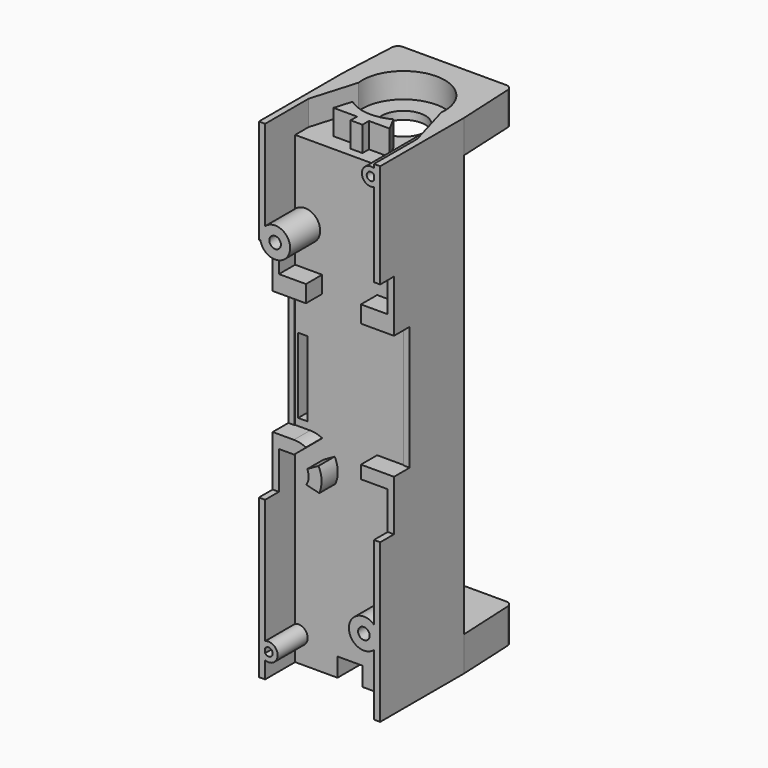
from build123d import *

# Parameters (mm, degrees)
F1_W           = 19.4
F1_H           = 5.4
F1_W_2         = 13
F1_H_2         = 3.4
F1_H_3         = 67.45
F1_R           = 2.4
F1_R_2         = 1.75
F2_DEPTH       = 13.5
F4_START       = -10
F4_DEPTH       = 17
F5_W           = 13
F5_H           = 3.4
F6_DEPTH       = 2.1
F7_DEPTH       = 2.25
F8_R           = 3.5
F9_DEPTH       = 7.5
F10_R          = 2
F11_DEPTH      = 7.5
F12_R          = 3.5
F13_DEPTH      = 4
F12_W          = 17.4
F12_H          = 6
F14_DEPTH      = 80
F15_W          = 3.989465184
F15_H          = 1.1423683461
F16_DEPTH      = 3
F17_W          = 2.7596634789
F17_H          = 19.85
F17_H_2        = 8.35
F17_W_2        = 3.1403365211
F17_H_3        = 8.1
F18_DEPTH      = 20
F19_W          = 1
F19_H          = 2.0696715653
F19_W_2        = 3.1403365211
F20_DEPTH      = 18.4
F21_DEPTH      = 25
F22_DEPTH      = 13.5
F23_W          = 8.7971314788
F23_H          = 3.2557382435
F24_DEPTH      = 80
F25_R          = 1.425
F25_R_2        = 0.65
F25_R_3        = 1.45
F26_DEPTH      = 21
F26_DEPTH_BACK = 6
F27_R          = 1.75
F27_R_2        = 0.925
F27_R_3        = 1.8673061799
F28_DEPTH      = 2.75
F29_W          = 1.5
F29_H          = 12
F30_DEPTH      = 21.001
F31_DEPTH      = 33.725
F32_R          = 6.2849648465
F33_DEPTH      = 2
F35_DEPTH      = 3.2403365211
F36_DEPTH      = 3.2403365211
F38_DEPTH      = 78.251


with BuildPart() as f2:
    # F1 (on Front) → F2 (new body, symmetric)
    with BuildSketch(Plane.XZ):
        with Locations((0, 75.55)):
            Rectangle(F1_W, F1_H)
        with Locations((0, 75.55)):
            Rectangle(F1_W_2, F1_H_2, mode=Mode.SUBTRACT)
        with Locations((0, 39.125)):
            Rectangle(F1_W, F1_H_3)
        with Locations((7.1, 11.6)):
            Circle(F1_R, mode=Mode.SUBTRACT)
        with Locations((-7.1, 62.05)):
            Circle(F1_R, mode=Mode.SUBTRACT)
        with Locations((-7.1, 62.05)):
            Circle(F1_R)
        with Locations((-7.1, 62.05)):
            Circle(F1_R_2, mode=Mode.SUBTRACT)
        with Locations((7.1, 11.6)):
            Circle(F1_R)
        with Locations((7.1, 11.6)):
            Circle(F1_R_2, mode=Mode.SUBTRACT)
        with Locations((0, 2.7)):
            Rectangle(F1_W, F1_H)
        with Locations((0, 2.7)):
            Rectangle(F1_W_2, F1_H_2, mode=Mode.SUBTRACT)
        with Locations((0, 2.7)):
            Rectangle(F1_W_2, F1_H_2)
        with Locations((0, 75.55)):
            Rectangle(F1_W_2, F1_H_2)
    extrude(amount=F2_DEPTH, both=True)

    # F1 (on Front) → F4 (cut)
    with BuildSketch(Plane.XZ.offset(F4_START)):
        with Locations((0, 2.7)):
            Rectangle(F1_W_2, F1_H_2)
        with Locations((0, 75.55)):
            Rectangle(F1_W_2, F1_H_2)
    extrude(amount=-F4_DEPTH, mode=Mode.SUBTRACT)

    # F5 (on face) → F6 (join)
    with BuildSketch(Plane(origin=(0, 13.5, 0), x_dir=(-1, 0, 0), z_dir=(0, 1, 0))):
        with Locations((0, 75.55)):
            Rectangle(F5_W, F5_H)
        with Locations((0, 2.7)):
            Rectangle(F5_W, F5_H)
    extrude(amount=-F6_DEPTH)

    # F5 (on face) → F7 (cut)
    with BuildSketch(Plane(origin=(0, 13.5, 0), x_dir=(-1, 0, 0), z_dir=(0, 1, 0))):
        with Locations((0, 75.55)):
            Rectangle(F5_W, F5_H)
        with Locations((0, 2.7)):
            Rectangle(F5_W, F5_H)
    extrude(amount=-F7_DEPTH, mode=Mode.SUBTRACT)

    # F8 (on face) → F9 (cut, symmetric)
    with BuildSketch(Plane.XY.offset(78.25)):
        with Locations((0, 3.3)):
            Circle(F8_R)
    extrude(amount=F9_DEPTH, both=True, mode=Mode.SUBTRACT)

    # F10 (on face) → F11 (cut, symmetric)
    with BuildSketch(Plane(origin=(0, 0, 0), x_dir=(1, 0, 0), z_dir=(0, 0, -1))):
        with Locations((0, -3.3)):
            Circle(F10_R)
    extrude(amount=F11_DEPTH, both=True, mode=Mode.SUBTRACT)

    # F12 (on face) → F13 (cut)
    with BuildSketch(Plane.XY.offset(78.25)):
        with BuildLine():
            Line((-6.5448551873, 2.4486066849), (-8.7, -4.8))
            Line((-8.7, -4.8), (-4.7295154072, -4.8))
            Line((-4.7295154072, -4.8), (-3.9035302168, -2.0218842383))
            ThreePointArc((-3.9035302168, -2.0218842383), (-5.6822980969, -0.0573037304), (-6.5448551873, 2.4486066849))
        make_face()
        with BuildLine():
            Line((8.7, -4.8), (6.5659687916, 2.6306317698))
            ThreePointArc((6.5659687916, 2.6306317698), (5.4611174799, -0.4062374277), (3.0469932229, -2.5545565417))
            Line((3.0469932229, -2.5545565417), (4.2667957023, -4.8))
            Line((4.2667957023, -4.8), (8.7, -4.8))
        make_face()
        Polygon((-4.7295154072, -4.8), (-8.7, -4.8), (-8.7, -7.5), (8.7, -7.5), (8.7, -4.8), (4.2667957023, -4.8), (0.95, -4.8), (0.95, -6.1), (-0.95, -6.1), (-0.95, -4.8), align=None)
        with BuildLine():
            ThreePointArc((6.6, 3.3), (-0.4265886565, 9.8861993682), (-6.5448551873, 2.4486066849))
            ThreePointArc((-6.5448551873, 2.4486066849), (-5.6822980969, -0.0573037304), (-3.9035302168, -2.0218842383))
            ThreePointArc((-3.9035302168, -2.0218842383), (-0.5043301014, -3.2807029373), (3.0469932229, -2.5545565417))
            ThreePointArc((3.0469932229, -2.5545565417), (5.4611174799, -0.4062374277), (6.5659687916, 2.6306317698))
            ThreePointArc((6.5659687916, 2.6306317698), (6.5914867073, 2.9648836207), (6.6, 3.3))
        make_face()
        with Locations((0, 3.3)):
            Circle(F12_R, mode=Mode.SUBTRACT)
    extrude(amount=-F13_DEPTH, mode=Mode.SUBTRACT)

    # F12 (on face) → F14 (cut)
    with BuildSketch(Plane.XY.offset(78.25)):
        with Locations((0, -10.5)):
            Rectangle(F12_W, F12_H)
    extrude(amount=-F14_DEPTH, mode=Mode.SUBTRACT)

    # F15 (on face) → F16 (cut)
    with BuildSketch(Plane(origin=(0, 0, 0), x_dir=(1, 0, 0), z_dir=(0, 0, -1))):
        with Locations((0.0731971226, 8.0711841731)):
            Rectangle(F15_W, F15_H)
        with BuildLine():
            ThreePointArc((1.9215354694, -2.7452915722), (0, -1.3), (-1.9215354694, -2.7452915722))
            Line((-1.9215354694, -2.7452915722), (1.9215354694, -2.7452915722))
        make_face()
        with BuildLine():
            Line((-1.9215354694, 7.5), (-1.9215354694, -2.7452915722))
            ThreePointArc((-1.9215354694, -2.7452915722), (0, -1.3), (1.9215354694, -2.7452915722))
            Line((1.9215354694, -2.7452915722), (2.0679297146, -2.7452915722))
            Line((2.0679297146, -2.7452915722), (2.0679297146, 7.5))
            Line((2.0679297146, 7.5), (-1.9215354694, 7.5))
        make_face()
    extrude(amount=-F16_DEPTH, mode=Mode.SUBTRACT)

    # F17 (on face) → F18 (cut, symmetric)
    with BuildSketch(Plane(origin=(-9.7, 0, 0), x_dir=(0, -1, 0), z_dir=(-1, 0, 0))):
        with Locations((12.1201682605, 43.325)):
            Rectangle(F17_W, F17_H)
        with Locations((12.1201682605, 57.425)):
            Rectangle(F17_W, F17_H_2)
        with Locations((9.1701682605, 43.325)):
            Rectangle(F17_W_2, F17_H)
        with Locations((12.1201682605, 29.35)):
            Rectangle(F17_W, F17_H_3)
    extrude(amount=F18_DEPTH, both=True, mode=Mode.SUBTRACT)

    # F19 (on face) → F20 (join, through all)
    with BuildSketch(Plane(origin=(-9.7, 0, 0), x_dir=(0, -1, 0), z_dir=(-1, 0, 0))):
        Polygon((6.6, 53.25), (7.6, 53.25), (10.7403365211, 53.25), (10.7403365211, 55.9618249536), (6.6, 55.9618249536), align=None)
        with Locations((7.1, 32.3651642174)):
            Rectangle(F19_W, F19_H)
        with Locations((9.1701682605, 32.3651642174)):
            Rectangle(F19_W_2, F19_H)
    extrude(amount=-F20_DEPTH)

    # F1 (on Front) → F21 (cut)
    with BuildSketch(Plane.XZ):
        with Locations((-7.1, 62.05)):
            Circle(F1_R_2)
    extrude(amount=F21_DEPTH, mode=Mode.SUBTRACT)

    # F1 (on Front) → F22 (join, through all)
    with BuildSketch(Plane.XZ):
        with Locations((7.1, 11.6)):
            Circle(F1_R)
        with Locations((7.1, 11.6)):
            Circle(F1_R_2, mode=Mode.SUBTRACT)
        with Locations((-7.1, 62.05)):
            Circle(F1_R)
        with Locations((-7.1, 62.05)):
            Circle(F1_R_2, mode=Mode.SUBTRACT)
    extrude(amount=F22_DEPTH)

    # F23 (on face) → F24 (cut)
    with BuildSketch(Plane(origin=(0, 0, 0), x_dir=(1, 0, 0), z_dir=(0, 0, -1))):
        with Locations((0.0165984966, 9.1278691217)):
            Rectangle(F23_W, F23_H)
    extrude(amount=-F24_DEPTH, mode=Mode.SUBTRACT)

    # F25 (on face) → F26 (join, two sides)
    with BuildSketch(Plane.XZ.offset(7.5)) as f26_sk:
        with Locations((8.2, 76.325)):
            Circle(F25_R)
        with Locations((8.2, 76.325)):
            Circle(F25_R_2, mode=Mode.SUBTRACT)
        with Locations((-8.15, 4.05)):
            Circle(F25_R_3)
        with Locations((-8.15, 4.05)):
            Circle(F25_R_2, mode=Mode.SUBTRACT)
    extrude(amount=-F26_DEPTH)
    extrude(f26_sk.sketch, amount=F26_DEPTH_BACK)

    # F27 (on face) → F28 (join)
    with BuildSketch(Plane.XZ.offset(13.5)):
        with Locations((-7.1, 62.05)):
            Circle(F27_R)
        with Locations((-7.1, 62.05)):
            Circle(F27_R_2, mode=Mode.SUBTRACT)
        with Locations((7.1, 11.6)):
            Circle(F27_R_3)
        with Locations((7.1, 11.6)):
            Circle(F27_R_2, mode=Mode.SUBTRACT)
    extrude(amount=-F28_DEPTH)

    # F29 (on face) → F30 (cut, through all)
    with BuildSketch(Plane.XZ.offset(7.5)):
        with Locations((-7.467607037, 40.5431138873)):
            Rectangle(F29_W, F29_H)
    extrude(amount=-F30_DEPTH, mode=Mode.SUBTRACT)

    # F3 (on offset) → F31 (cut, symmetric)
    with BuildSketch(Plane.XY.offset(39.25)):
        with BuildLine():
            ThreePointArc((9.7, 3.3), (0, 13), (-9.7, 3.3))
            Line((-9.7, 3.3), (9.7, 3.3))
        make_face()
        with BuildLine():
            Line((-9.7, 13.5), (-9.7, 3.3))
            ThreePointArc((-9.7, 3.3), (0, 13), (9.7, 3.3))
            Line((9.7, 3.3), (9.7, 13.5))
            Line((9.7, 13.5), (-9.7, 13.5))
        make_face()
        with BuildLine():
            Line((9.7, 3.3), (-9.7, 3.3))
            ThreePointArc((-9.7, 3.3), (0, -6.4), (9.7, 3.3))
        make_face()
    extrude(amount=F31_DEPTH, both=True, mode=Mode.SUBTRACT)

    # F32 (on face) → F33 (cut)
    with BuildSketch(Plane(origin=(0, 0, 0), x_dir=(1, 0, 0), z_dir=(0, 0, -1))):
        with Locations((0, -3.3)):
            Circle(F32_R)
    extrude(amount=-F33_DEPTH, mode=Mode.SUBTRACT)

    # F34 (on face) → F35 (cut, through all)
    with BuildSketch(Plane.XZ.offset(7.5)):
        Polygon((-4.3819672428, 33.6735062301), (-7.4980124951, 33.6735062301), (-7.4980124951, 33.4), (-6.309012777, 33.4), (-4.3819672428, 33.4), align=None)
        Polygon((-4.3819672428, 31.3303284347), (-4.3819672428, 32.9217889321), (-6.2805607904, 31.3303284347), align=None)
        with BuildLine():
            ThreePointArc((-2.2529312209, 27.2007325665), (-1.8847040899, 29.114246198), (-2.3738502676, 31.000475679))
            Line((-2.3738502676, 31.000475679), (-4.1782804969, 29.9808483851))
            ThreePointArc((-4.1782804969, 29.9808483851), (-3.9562194224, 28.8347732192), (-4.3113791264, 27.7227206164))
            Line((-4.3113791264, 27.7227206164), (-2.2529312209, 27.2007325665))
        make_face()
        with BuildLine():
            ThreePointArc((-2.3738502676, 31.000475679), (-3.2077114124, 32.1319734864), (-4.3542633766, 32.9450111793))
            Line((-4.3542633766, 32.9450111793), (-4.3819672428, 32.9217889321))
            Line((-4.3819672428, 32.9217889321), (-4.3819672428, 31.3303284347))
            Line((-4.3819672428, 31.3303284347), (-4.3819672428, 30.8272019029))
            Line((-4.3819672428, 30.8272019029), (-4.8535134819, 30.8272019029))
            ThreePointArc((-4.8535134819, 30.8272019029), (-4.4666385487, 30.443324235), (-4.1782804969, 29.9808483851))
            Line((-4.1782804969, 29.9808483851), (-2.3738502676, 31.000475679))
        make_face()
        with BuildLine():
            Line((-4.3819672428, 31.3303284347), (-6.2805607904, 31.3303284347))
            Line((-6.2805607904, 31.3303284347), (-6.2807627766, 31.3301591235))
            ThreePointArc((-6.2807627766, 31.3301591235), (-5.6213249589, 31.2277705376), (-5.0170200476, 30.9446500116))
            ThreePointArc((-5.0170200476, 30.9446500116), (-4.9340121876, 30.8876725294), (-4.8535134819, 30.8272019029))
            Line((-4.8535134819, 30.8272019029), (-4.3819672428, 30.8272019029))
            Line((-4.3819672428, 30.8272019029), (-4.3819672428, 31.3303284347))
        make_face()
        with BuildLine():
            ThreePointArc((-6.309012777, 31.3303284347), (-6.9249139857, 31.2484316241), (-7.4980124951, 31.0084326969))
            Line((-7.4980124951, 31.0084326969), (-7.4980124951, 30.8272019029))
            Line((-7.4980124951, 30.8272019029), (-4.8535134819, 30.8272019029))
            ThreePointArc((-4.8535134819, 30.8272019029), (-4.9340121876, 30.8876725294), (-5.0170200476, 30.9446500116))
            ThreePointArc((-5.0170200476, 30.9446500116), (-5.6213249589, 31.2277705376), (-6.2807627766, 31.3301591235))
            ThreePointArc((-6.2807627766, 31.3301591235), (-6.2948875231, 31.3302861065), (-6.309012777, 31.3303284347))
        make_face()
        with BuildLine():
            Line((-6.309012777, 31.3303284347), (-7.4980124951, 31.3303284347))
            Line((-7.4980124951, 31.3303284347), (-7.4980124951, 31.0084326969))
            ThreePointArc((-7.4980124951, 31.0084326969), (-6.9249139857, 31.2484316241), (-6.309012777, 31.3303284347))
        make_face()
        with BuildLine():
            Line((-7.4980124951, 30.8272019029), (-7.4980124951, 31.0084326969))
            ThreePointArc((-7.4980124951, 31.0084326969), (-8.0008898937, 27.3325920712), (-4.3113791264, 27.7227206164))
            ThreePointArc((-4.3113791264, 27.7227206164), (-3.9562194224, 28.8347732192), (-4.1782804969, 29.9808483851))
            ThreePointArc((-4.1782804969, 29.9808483851), (-4.4666385487, 30.443324235), (-4.8535134819, 30.8272019029))
            Line((-4.8535134819, 30.8272019029), (-7.4980124951, 30.8272019029))
        make_face()
        with BuildLine():
            Line((-4.3819672428, 32.9585270347), (-4.3819672428, 33.4))
            Line((-4.3819672428, 33.4), (-6.309012777, 33.4))
            ThreePointArc((-6.309012777, 33.4), (-5.3205287268, 33.288220425), (-4.3819672428, 32.9585270347))
        make_face()
    extrude(amount=F35_DEPTH, mode=Mode.SUBTRACT)

    # F34 (on face) → F36 (join, through all)
    with BuildSketch(Plane.XZ.offset(7.5)):
        with BuildLine():
            ThreePointArc((-2.2529312209, 27.2007325665), (-1.8847040899, 29.114246198), (-2.3738502676, 31.000475679))
            Line((-2.3738502676, 31.000475679), (-4.1782804969, 29.9808483851))
            ThreePointArc((-4.1782804969, 29.9808483851), (-3.9562194224, 28.8347732192), (-4.3113791264, 27.7227206164))
            Line((-4.3113791264, 27.7227206164), (-2.2529312209, 27.2007325665))
        make_face()
    extrude(amount=F36_DEPTH)

    # F37 (on face) → F38 (cut, through all)
    with BuildSketch(Plane(origin=(0, 0, 0), x_dir=(1, 0, 0), z_dir=(0, 0, -1))):
        with BuildLine():
            Line((-9.2466195677, -12.5489608186), (-9.7, -3.3))
            Line((-9.7, -3.3), (-9.7, -13.5))
            Line((-9.7, -13.5), (-8.2478188678, -13.5))
            ThreePointArc((-8.2478188678, -13.5), (-8.937398153, -13.2242101969), (-9.2466195677, -12.5489608186))
        make_face()
        with BuildLine():
            ThreePointArc((9.2466195677, -12.5489608186), (8.937398153, -13.2242101969), (8.2478188678, -13.5))
            Line((8.2478188678, -13.5), (9.7, -13.5))
            Line((9.7, -13.5), (9.7, -3.3))
            Line((9.7, -3.3), (9.2466195677, -12.5489608186))
        make_face()
    extrude(amount=-F38_DEPTH, mode=Mode.SUBTRACT)


solid = f2.part
